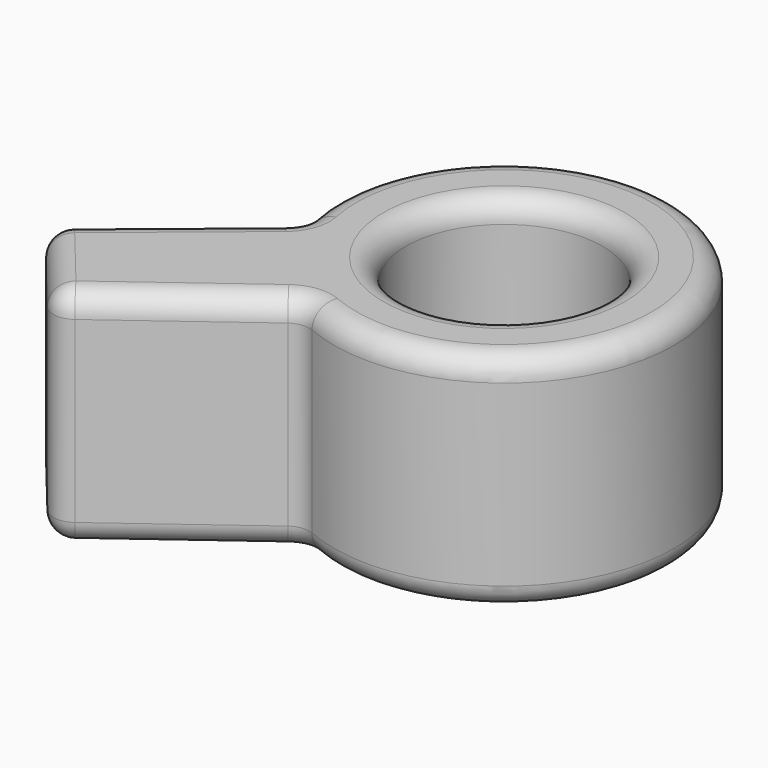
from build123d import *

# Parameters (mm, degrees)
F0_R     = 22.03
F1_DEPTH = 50
F2_R     = 5
F3_T     = -2.5


with BuildPart() as f1:
    # F0 (on Top) → F1 (new body)
    with BuildSketch(Plane.XY):
        with BuildLine():
            ThreePointArc((19.111431778, -6.8960115293), (56.4366245885, -5.6218490797), (74.7410013376, 26.9318496366))
            ThreePointArc((74.7410013376, 26.9318496366), (31.369006979, 64.6653370911), (0, 16.4892914742))
            ThreePointArc((0, 16.4892914742), (7.1396320987, 2.8221168918), (19.111431778, -6.8960115293))
        make_face()
        with Locations((36.6410013376, 26.9318496366)):
            Circle(F0_R, mode=Mode.SUBTRACT)
        with BuildLine():
            ThreePointArc((19.111431778, -6.8960115293), (7.1396320987, 2.8221168918), (0, 16.4892914742))
            Line((0, 16.4892914742), (-34.7932870747, -12.0488790092))
            Line((-34.7932870747, -12.0488790092), (-17.0362032183, -33.6980354112))
            Line((-17.0362032183, -33.6980354112), (19.111431778, -6.8960115293))
        make_face()
    extrude(amount=F1_DEPTH)

    # F2
    f2_edges = [f1.edges().sort_by_distance(p)[0] for p in [
        (66.142371, 51.041582, 50),
        (14.611001, 26.93185, 50),
        (-17.396644, 2.220206, 50),
        (1.037614, -20.297023, 50),
        (0, 16.489291, 25),
        (-34.793287, -12.048879, 25),
        (19.111432, -6.896012, 25),
        (-17.036203, -33.698035, 25),
        (-25.914745, -22.873457, 0),
        (-25.914745, -22.873457, 50),
        (66.142371, 51.041582, 0),
        (14.611001, 26.93185, 0),
        (-17.396644, 2.220206, 0),
        (1.037614, -20.297023, 0),
    ]]
    fillet(f2_edges, radius=F2_R)

    # F3 (hollow: no face is removed)
    offset(amount=F3_T, mode=Mode.SUBTRACT)


solid = f1.part
